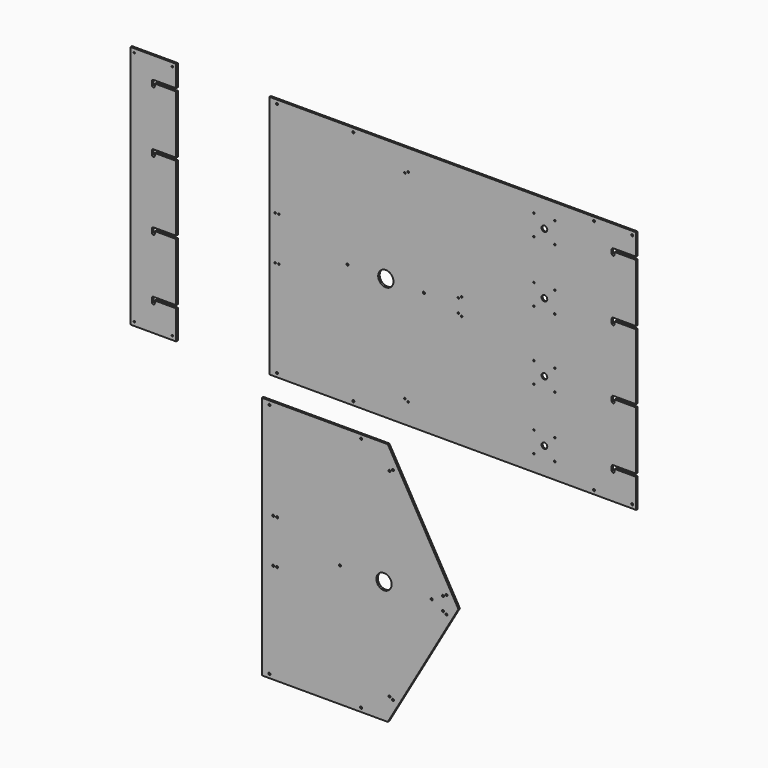
from build123d import *

# Parameters (mm, degrees)
F1_DEPTH     = 6.35
F3_D         = 5.1054
F3_DEPTH     = 26.0604
F3_TIP       = 1.5338169022
F4_W         = 4.7625
F4_H         = 4.7625
F5_DEPTH     = 25.4
F7_D         = 6.7564
F7_DEPTH     = 26.0604
F7_TIP       = 2.0298273432
F9_DEPTH     = 6.35
F10_R        = 9.525
F11_DEPTH    = 25.4
F12_D        = 5.1054
F12_DEPTH    = 26.0604
F12_TIP      = 1.5338169022
F13_R        = 38.1
F14_DEPTH    = 2.032
F6_R         = 25.4
F1_FACE1_R   = 3.3782
F1_FACE1_R_2 = 2.5527
F1_FACE1_R_3 = 38.1
F15_DEPTH    = 25.4
F16_D        = 5.1054
F16_DEPTH    = 26.0604
F16_TIP      = 1.5338169022
F18_D        = 6.7564
F19_R        = 25.4
F19_W        = 25.4
F19_H        = 812.8
F20_DEPTH    = 6.35
F21_D        = 6.7564
F21_DEPTH    = 26.0604
F21_TIP      = 2.0298273432


# Not quite as in the source:
# - a feature names something its author has since deleted; it is built from what else it names


with BuildPart() as f1:
    # F0 (on Front) → F1 (new body)
    with BuildSketch(Plane.XZ):
        Polygon((0, 47.625), (0, 0), (1219.2, 0), (1219.2, 812.8), (53.975, 812.8), (0, 812.8), (0, 508), (0, 406.4), (0, 304.8), (0, 104.775), align=None)
    extrude(amount=-F1_DEPTH)

    # F3
    with Locations(Plane.XZ):
        with Locations((450.3940905122, 76.2), (461.3926131403, 69.85), (639.1926131403, 377.8086335857), (628.1940905122, 384.1586335857), (639.1926131403, 434.9913664143), (628.1940905122, 428.6413664143), (461.3926131403, 742.95), (450.3940905122, 736.6), (31.75, 333.375), (19.05, 479.425), (31.75, 479.425), (19.05, 333.375)):
            Hole(F3_D / 2, depth=F3_DEPTH)
            with Locations((0, 0, -(F3_DEPTH + F3_TIP / 2))):  # 118° drill point
                Cone(0, F3_D / 2, F3_TIP, mode=Mode.SUBTRACT)

    # F4 (on face) → F5 (cut)
    with BuildSketch(Plane.XZ):
        with Locations((1145.38125, 734.21875)):
            Rectangle(F4_W, F4_H)
        with BuildLine():
            Line((1143, 736.6), (1147.7625, 736.6))
            ThreePointArc((1147.7625, 736.6), (1146.3675960454, 739.9675960454), (1143, 741.3625))
            ThreePointArc((1143, 741.3625), (1139.6324039546, 739.9675960454), (1138.2375, 736.6))
            ThreePointArc((1138.2375, 736.6), (1139.6324039546, 733.2324039546), (1143, 731.8375))
            Line((1143, 731.8375), (1143, 736.6))
        make_face()
        with BuildLine():
            ThreePointArc((1143, 741.3625), (1146.3675960454, 739.9675960454), (1147.7625, 736.6))
            Line((1147.7625, 736.6), (1147.7625, 731.8375))
            Line((1147.7625, 731.8375), (1219.2, 731.8375))
            ThreePointArc((1219.2, 731.8375), (1223.9625, 736.6), (1219.2, 741.3625))
            Line((1219.2, 741.3625), (1143, 741.3625))
        make_face()
        with BuildLine():
            Line((1147.7625, 723.9), (1147.7625, 731.8375))
            Line((1147.7625, 731.8375), (1143, 731.8375))
            ThreePointArc((1143, 731.8375), (1139.6324039546, 733.2324039546), (1138.2375, 736.6))
            Line((1138.2375, 736.6), (1138.2375, 723.9))
            ThreePointArc((1138.2375, 723.9), (1143, 719.1375), (1147.7625, 723.9))
        make_face()
        with Locations((1145.38125, 531.01875)):
            Rectangle(F4_W, F4_H)
        with BuildLine():
            Line((1143, 533.4), (1147.7625, 533.4))
            ThreePointArc((1147.7625, 533.4), (1146.3675960454, 536.7675960454), (1143, 538.1625))
            ThreePointArc((1143, 538.1625), (1139.6324039546, 536.7675960454), (1138.2375, 533.4))
            ThreePointArc((1138.2375, 533.4), (1139.6324039546, 530.0324039546), (1143, 528.6375))
            Line((1143, 528.6375), (1143, 533.4))
        make_face()
        with BuildLine():
            ThreePointArc((1143, 538.1625), (1146.3675960454, 536.7675960454), (1147.7625, 533.4))
            Line((1147.7625, 533.4), (1147.7625, 528.6375))
            Line((1147.7625, 528.6375), (1219.2, 528.6375))
            ThreePointArc((1219.2, 528.6375), (1223.9625, 533.4), (1219.2, 538.1625))
            Line((1219.2, 538.1625), (1143, 538.1625))
        make_face()
        with BuildLine():
            Line((1147.7625, 520.7), (1147.7625, 528.6375))
            Line((1147.7625, 528.6375), (1143, 528.6375))
            ThreePointArc((1143, 528.6375), (1139.6324039546, 530.0324039546), (1138.2375, 533.4))
            Line((1138.2375, 533.4), (1138.2375, 520.7))
            ThreePointArc((1138.2375, 520.7), (1143, 515.9375), (1147.7625, 520.7))
        make_face()
        with Locations((1145.38125, 302.41875)):
            Rectangle(F4_W, F4_H)
        with BuildLine():
            Line((1143, 304.8), (1147.7625, 304.8))
            ThreePointArc((1147.7625, 304.8), (1146.3675960454, 308.1675960454), (1143, 309.5625))
            ThreePointArc((1143, 309.5625), (1139.6324039546, 308.1675960454), (1138.2375, 304.8))
            ThreePointArc((1138.2375, 304.8), (1139.6324039546, 301.4324039546), (1143, 300.0375))
            Line((1143, 300.0375), (1143, 304.8))
        make_face()
        with BuildLine():
            ThreePointArc((1143, 309.5625), (1146.3675960454, 308.1675960454), (1147.7625, 304.8))
            Line((1147.7625, 304.8), (1147.7625, 300.0375))
            Line((1147.7625, 300.0375), (1219.2, 300.0375))
            ThreePointArc((1219.2, 300.0375), (1223.9625, 304.8), (1219.2, 309.5625))
            Line((1219.2, 309.5625), (1143, 309.5625))
        make_face()
        with BuildLine():
            Line((1147.7625, 292.1), (1147.7625, 300.0375))
            Line((1147.7625, 300.0375), (1143, 300.0375))
            ThreePointArc((1143, 300.0375), (1139.6324039546, 301.4324039546), (1138.2375, 304.8))
            Line((1138.2375, 304.8), (1138.2375, 292.1))
            ThreePointArc((1138.2375, 292.1), (1143, 287.3375), (1147.7625, 292.1))
        make_face()
        with Locations((1145.38125, 99.21875)):
            Rectangle(F4_W, F4_H)
        with BuildLine():
            Line((1143, 101.6), (1147.7625, 101.6))
            ThreePointArc((1147.7625, 101.6), (1146.3675960454, 104.9675960454), (1143, 106.3625))
            ThreePointArc((1143, 106.3625), (1139.6324039546, 104.9675960454), (1138.2375, 101.6))
            ThreePointArc((1138.2375, 101.6), (1139.6324039546, 98.2324039546), (1143, 96.8375))
            Line((1143, 96.8375), (1143, 101.6))
        make_face()
        with BuildLine():
            ThreePointArc((1143, 106.3625), (1146.3675960454, 104.9675960454), (1147.7625, 101.6))
            Line((1147.7625, 101.6), (1147.7625, 96.8375))
            Line((1147.7625, 96.8375), (1219.2, 96.8375))
            ThreePointArc((1219.2, 96.8375), (1223.9625, 101.6), (1219.2, 106.3625))
            Line((1219.2, 106.3625), (1143, 106.3625))
        make_face()
        with BuildLine():
            Line((1147.7625, 88.9), (1147.7625, 96.8375))
            Line((1147.7625, 96.8375), (1143, 96.8375))
            ThreePointArc((1143, 96.8375), (1139.6324039546, 98.2324039546), (1138.2375, 101.6))
            Line((1138.2375, 101.6), (1138.2375, 88.9))
            ThreePointArc((1138.2375, 88.9), (1143, 84.1375), (1147.7625, 88.9))
        make_face()
    extrude(amount=-F5_DEPTH, mode=Mode.SUBTRACT)

    # F7
    with Locations(Plane.XZ):
        with Locations((25.4, 800.1), (279.4, 800.1), (25.4, 12.7), (279.4, 12.7), (260.0351493987, 406.4), (514.0351493987, 406.4)):
            Hole(F7_D / 2, depth=F7_DEPTH)
            with Locations((0, 0, -(F7_DEPTH + F7_TIP / 2))):  # 118° drill point
                Cone(0, F7_D / 2, F7_TIP, mode=Mode.SUBTRACT)

    # F10 (on face) → F11 (cut)
    with BuildSketch(Plane(origin=(0, 6.35, 0), x_dir=(-1, 0, 0), z_dir=(0, 1, 0))):
        with Locations((-914.4, 723.9)):
            Circle(F10_R)
        with Locations((-914.4, 520.7)):
            Circle(F10_R)
        with Locations((-914.4, 292.1)):
            Circle(F10_R)
        with Locations((-914.4, 88.9)):
            Circle(F10_R)
    extrude(amount=-F11_DEPTH, mode=Mode.SUBTRACT)

    # F12
    with Locations(Plane(origin=(0, 6.35, 0), x_dir=(-1, 0, 0), z_dir=(0, 1, 0))):
        with Locations((-949.2074727253, 689.0925272747), (-879.5925272747, 689.0925272747), (-879.5925272747, 758.7074727253), (-949.2074727253, 758.7074727253), (-949.2074727253, 555.5074727253), (-879.5925272747, 555.5074727253), (-879.5925272747, 485.8925272747), (-949.2074727253, 485.8925272747), (-949.2074727253, 326.9074727253), (-879.5925272747, 326.9074727253), (-879.5925272747, 257.2925272747), (-949.2074727253, 257.2925272747), (-879.5925272747, 123.7074727253), (-949.2074727253, 123.7074727253), (-949.2074727253, 54.0925272747), (-879.5925272747, 54.0925272747)):
            Hole(F12_D / 2, depth=F12_DEPTH)
            with Locations((0, 0, -(F12_DEPTH + F12_TIP / 2))):  # 118° drill point
                Cone(0, F12_D / 2, F12_TIP, mode=Mode.SUBTRACT)

    # F13 (on face) → F14 (cut)
    with BuildSketch(Plane(origin=(0, 6.35, 0), x_dir=(-1, 0, 0), z_dir=(0, 1, 0))):
        with Locations((-914.4, 723.9)):
            Circle(F13_R)
        with Locations((-914.4, 520.7)):
            Circle(F13_R)
        with Locations((-914.4, 292.1)):
            Circle(F13_R)
        with Locations((-914.4, 88.9)):
            Circle(F13_R)
    extrude(amount=-F14_DEPTH, mode=Mode.SUBTRACT)

    # F6 (on face) + F1_face1 (on face) → F15 (cut)
    with BuildSketch(Plane.XZ):
        with Locations((387.0351493987, 406.4)):
            Circle(F6_R)
    with BuildSketch(Plane(origin=(607.7331419977, 6.35, 406.3597077794), x_dir=(1, 0, 0), z_dir=(0, 1, 0))):
        with BuildLine():
            Line((-607.7331419977, 406.3597077794), (-607.7331419977, -406.4402922206))
            Line((-607.7331419977, -406.4402922206), (611.4668580023, -406.4402922206))
            Line((611.4668580023, -406.4402922206), (611.4668580023, -335.0027922206))
            Line((611.4668580023, -335.0027922206), (535.2668580023, -335.0027922206))
            ThreePointArc((535.2668580023, -335.0027922206), (531.8992619569, -333.607888266), (530.5043580023, -330.2402922206))
            Line((530.5043580023, -330.2402922206), (530.5043580023, -317.5402922206))
            ThreePointArc((530.5043580023, -317.5402922206), (535.2668580023, -312.7777922206), (540.0293580023, -317.5402922206))
            Line((540.0293580023, -317.5402922206), (540.0293580023, -325.4777922206))
            Line((540.0293580023, -325.4777922206), (611.4668580023, -325.4777922206))
            Line((611.4668580023, -325.4777922206), (611.4668580023, -131.8027922206))
            Line((611.4668580023, -131.8027922206), (535.2668580023, -131.8027922206))
            ThreePointArc((535.2668580023, -131.8027922206), (531.8992619569, -130.407888266), (530.5043580023, -127.0402922206))
            Line((530.5043580023, -127.0402922206), (530.5043580023, -114.3402922206))
            ThreePointArc((530.5043580023, -114.3402922206), (535.2668580023, -109.5777922206), (540.0293580023, -114.3402922206))
            Line((540.0293580023, -114.3402922206), (540.0293580023, -122.2777922206))
            Line((540.0293580023, -122.2777922206), (611.4668580023, -122.2777922206))
            Line((611.4668580023, -122.2777922206), (611.4668580023, 96.7972077794))
            Line((611.4668580023, 96.7972077794), (535.2668580023, 96.7972077794))
            ThreePointArc((535.2668580023, 96.7972077794), (531.8992619569, 98.192111734), (530.5043580023, 101.5597077794))
            Line((530.5043580023, 101.5597077794), (530.5043580023, 114.2597077794))
            ThreePointArc((530.5043580023, 114.2597077794), (535.2668580023, 119.0222077794), (540.0293580023, 114.2597077794))
            Line((540.0293580023, 114.2597077794), (540.0293580023, 106.3222077794))
            Line((540.0293580023, 106.3222077794), (611.4668580023, 106.3222077794))
            Line((611.4668580023, 106.3222077794), (611.4668580023, 299.9972077794))
            Line((611.4668580023, 299.9972077794), (535.2668580023, 299.9972077794))
            ThreePointArc((535.2668580023, 299.9972077794), (531.8992619569, 301.392111734), (530.5043580023, 304.7597077794))
            Line((530.5043580023, 304.7597077794), (530.5043580023, 317.4597077794))
            ThreePointArc((530.5043580023, 317.4597077794), (535.2668580023, 322.2222077794), (540.0293580023, 317.4597077794))
            Line((540.0293580023, 317.4597077794), (540.0293580023, 309.5222077794))
            Line((540.0293580023, 309.5222077794), (611.4668580023, 309.5222077794))
            Line((611.4668580023, 309.5222077794), (611.4668580023, 406.3597077794))
            Line((611.4668580023, 406.3597077794), (-607.7331419977, 406.3597077794))
        make_face()
        with Locations((-582.3331419977, 393.6597077794)):
            Circle(F1_FACE1_R, mode=Mode.SUBTRACT)
        with Locations((-328.3331419977, 393.6597077794)):
            Circle(F1_FACE1_R, mode=Mode.SUBTRACT)
        with Locations((-157.3390514855, 330.1597077794)):
            Circle(F1_FACE1_R_2, mode=Mode.SUBTRACT)
        with Locations((-146.3405288574, 336.5097077794)):
            Circle(F1_FACE1_R_2, mode=Mode.SUBTRACT)
        with Locations((-588.6831419977, 72.9847077794)):
            Circle(F1_FACE1_R_2, mode=Mode.SUBTRACT)
        with Locations((-575.9831419977, 72.9847077794)):
            Circle(F1_FACE1_R_2, mode=Mode.SUBTRACT)
        with Locations((-347.6979925991, -0.0402922206)):
            Circle(F1_FACE1_R, mode=Mode.SUBTRACT)
        with Locations((271.859385277, 352.2671805047)):
            Circle(F1_FACE1_R_2, mode=Mode.SUBTRACT)
        with Locations((341.4743307275, 352.2671805047)):
            Circle(F1_FACE1_R_2, mode=Mode.SUBTRACT)
        with Locations((306.6668580023, 317.4597077794)):
            Circle(F1_FACE1_R_3, mode=Mode.SUBTRACT)
        with Locations((271.859385277, 282.6522350541)):
            Circle(F1_FACE1_R_2, mode=Mode.SUBTRACT)
        with Locations((341.4743307275, 282.6522350541)):
            Circle(F1_FACE1_R_2, mode=Mode.SUBTRACT)
        with Locations((-93.6979925991, -0.0402922206)):
            Circle(F1_FACE1_R, mode=Mode.SUBTRACT)
        with Locations((31.4594711426, 28.5510741937)):
            Circle(F1_FACE1_R_2, mode=Mode.SUBTRACT)
        with Locations((20.4609485145, 22.2010741937)):
            Circle(F1_FACE1_R_2, mode=Mode.SUBTRACT)
        with Locations((271.859385277, 149.0671805047)):
            Circle(F1_FACE1_R_2, mode=Mode.SUBTRACT)
        with Locations((341.4743307275, 149.0671805047)):
            Circle(F1_FACE1_R_2, mode=Mode.SUBTRACT)
        with Locations((306.6668580023, 114.2597077794)):
            Circle(F1_FACE1_R_3, mode=Mode.SUBTRACT)
        with Locations((271.859385277, 79.4522350541)):
            Circle(F1_FACE1_R_2, mode=Mode.SUBTRACT)
        with Locations((341.4743307275, 79.4522350541)):
            Circle(F1_FACE1_R_2, mode=Mode.SUBTRACT)
        with Locations((-588.6831419977, -73.0652922206)):
            Circle(F1_FACE1_R_2, mode=Mode.SUBTRACT)
        with Locations((-575.9831419977, -73.0652922206)):
            Circle(F1_FACE1_R_2, mode=Mode.SUBTRACT)
        with Locations((-582.3331419977, -393.7402922206)):
            Circle(F1_FACE1_R, mode=Mode.SUBTRACT)
        with Locations((-328.3331419977, -393.7402922206)):
            Circle(F1_FACE1_R, mode=Mode.SUBTRACT)
        with Locations((-157.3390514855, -330.2402922206)):
            Circle(F1_FACE1_R_2, mode=Mode.SUBTRACT)
        with Locations((-146.3405288574, -336.5902922206)):
            Circle(F1_FACE1_R_2, mode=Mode.SUBTRACT)
        with Locations((20.4609485145, -22.2816586348)):
            Circle(F1_FACE1_R_2, mode=Mode.SUBTRACT)
        with Locations((31.4594711426, -28.6316586348)):
            Circle(F1_FACE1_R_2, mode=Mode.SUBTRACT)
        with Locations((271.859385277, -79.5328194953)):
            Circle(F1_FACE1_R_2, mode=Mode.SUBTRACT)
        with Locations((341.4743307275, -79.5328194953)):
            Circle(F1_FACE1_R_2, mode=Mode.SUBTRACT)
        with Locations((306.6668580023, -114.3402922206)):
            Circle(F1_FACE1_R_3, mode=Mode.SUBTRACT)
        with Locations((271.859385277, -149.1477649459)):
            Circle(F1_FACE1_R_2, mode=Mode.SUBTRACT)
        with Locations((341.4743307275, -149.1477649459)):
            Circle(F1_FACE1_R_2, mode=Mode.SUBTRACT)
        with Locations((271.859385277, -282.7328194953)):
            Circle(F1_FACE1_R_2, mode=Mode.SUBTRACT)
        with Locations((341.4743307275, -282.7328194953)):
            Circle(F1_FACE1_R_2, mode=Mode.SUBTRACT)
        with Locations((306.6668580023, -317.5402922206)):
            Circle(F1_FACE1_R_3, mode=Mode.SUBTRACT)
        with Locations((271.859385277, -352.3477649459)):
            Circle(F1_FACE1_R_2, mode=Mode.SUBTRACT)
        with Locations((341.4743307275, -352.3477649459)):
            Circle(F1_FACE1_R_2, mode=Mode.SUBTRACT)
    extrude(amount=-F15_DEPTH, dir=(0, -1, 0), mode=Mode.SUBTRACT)

    # F18 (through all)
    with Locations(Plane.XZ):
        with Locations((1206.5, 800.1), (1079.5, 800.1), (1206.5, 12.7), (1079.5, 12.7)):
            Hole(F18_D / 2)


with BuildPart() as f9:
    # F8 (on Front) → F9 (new body)
    with BuildSketch(Plane.XZ):
        with BuildLine():
            Line((-457.2, 0), (-304.8, 0))
            Line((-304.8, 0), (-304.8, 96.8375))
            Line((-304.8, 96.8375), (-376.2375, 96.8375))
            Line((-376.2375, 96.8375), (-376.2375, 88.9))
            ThreePointArc((-376.2375, 88.9), (-381, 84.1375), (-385.7625, 88.9))
            Line((-385.7625, 88.9), (-385.7625, 101.6))
            ThreePointArc((-385.7625, 101.6), (-384.3675960454, 104.9675960454), (-381, 106.3625))
            Line((-381, 106.3625), (-304.8, 106.3625))
            Line((-304.8, 106.3625), (-304.8, 300.0375))
            Line((-304.8, 300.0375), (-376.2375, 300.0375))
            Line((-376.2375, 300.0375), (-376.2375, 292.1))
            ThreePointArc((-376.2375, 292.1), (-381, 287.3375), (-385.7625, 292.1))
            Line((-385.7625, 292.1), (-385.7625, 304.8))
            ThreePointArc((-385.7625, 304.8), (-384.3675960454, 308.1675960454), (-381, 309.5625))
            Line((-381, 309.5625), (-304.8, 309.5625))
            Line((-304.8, 309.5625), (-304.8, 528.6375))
            Line((-304.8, 528.6375), (-376.2375, 528.6375))
            Line((-376.2375, 528.6375), (-376.2375, 520.7))
            ThreePointArc((-376.2375, 520.7), (-381, 515.9375), (-385.7625, 520.7))
            Line((-385.7625, 520.7), (-385.7625, 533.4))
            ThreePointArc((-385.7625, 533.4), (-384.3675960454, 536.7675960454), (-381, 538.1625))
            Line((-381, 538.1625), (-304.8, 538.1625))
            Line((-304.8, 538.1625), (-304.8, 731.8375))
            Line((-304.8, 731.8375), (-376.2375, 731.8375))
            Line((-376.2375, 731.8375), (-376.2375, 723.9))
            ThreePointArc((-376.2375, 723.9), (-381, 719.1375), (-385.7625, 723.9))
            Line((-385.7625, 723.9), (-385.7625, 736.6))
            ThreePointArc((-385.7625, 736.6), (-384.3675960454, 739.9675960454), (-381, 741.3625))
            Line((-381, 741.3625), (-304.8, 741.3625))
            Line((-304.8, 741.3625), (-304.8, 812.8))
            Line((-304.8, 812.8), (-457.2, 812.8))
            Line((-457.2, 812.8), (-457.2, 0))
        make_face()
    extrude(amount=F9_DEPTH)

    # F16
    with Locations(Plane(origin=(0, 0, 0), x_dir=(1, 0, 0), z_dir=(0, 1, 0))):
        with Locations((-444.5, -800.1), (-317.5, -800.1), (-317.5, -12.7), (-444.5, -12.7)):
            Hole(F16_D / 2, depth=F16_DEPTH)
            with Locations((0, 0, -(F16_DEPTH + F16_TIP / 2))):  # 118° drill point
                Cone(0, F16_D / 2, F16_TIP, mode=Mode.SUBTRACT)


with BuildPart() as f20:
    # F19 (on Front) → F20 (new body)
    with BuildSketch(Plane.XZ):
        Polygon((393.7, -76.2), (0, -76.2), (0, -889), (393.7, -889), (628.3351493987, -482.6), align=None)
        with Locations((381, -482.6)):
            Circle(F19_R, mode=Mode.SUBTRACT)
        with Locations((-12.7, -482.6)):
            Rectangle(F19_W, F19_H)
    extrude(amount=-F20_DEPTH)

    # F21
    with Locations(Plane.XZ):
        with Locations((25.4, -409.575), (12.7, -409.575), (25.4, -555.625), (12.7, -555.625), (399.5940905122, -812.8), (410.5926131403, -819.15), (577.3940905122, -504.8413664143), (588.3926131403, -511.1913664143), (577.3940905122, -460.3586335857), (588.3926131403, -454.0086335857), (399.5940905122, -152.4), (410.5926131403, -146.05), (304.8, -876.3), (0, -876.3), (304.8, -88.9), (0, -88.9), (234.6452, -482.6), (539.4452, -482.6)):
            Hole(F21_D / 2, depth=F21_DEPTH)
            with Locations((0, 0, -(F21_DEPTH + F21_TIP / 2))):  # 118° drill point
                Cone(0, F21_D / 2, F21_TIP, mode=Mode.SUBTRACT)


solid = Compound([f1.part, f9.part, f20.part])
